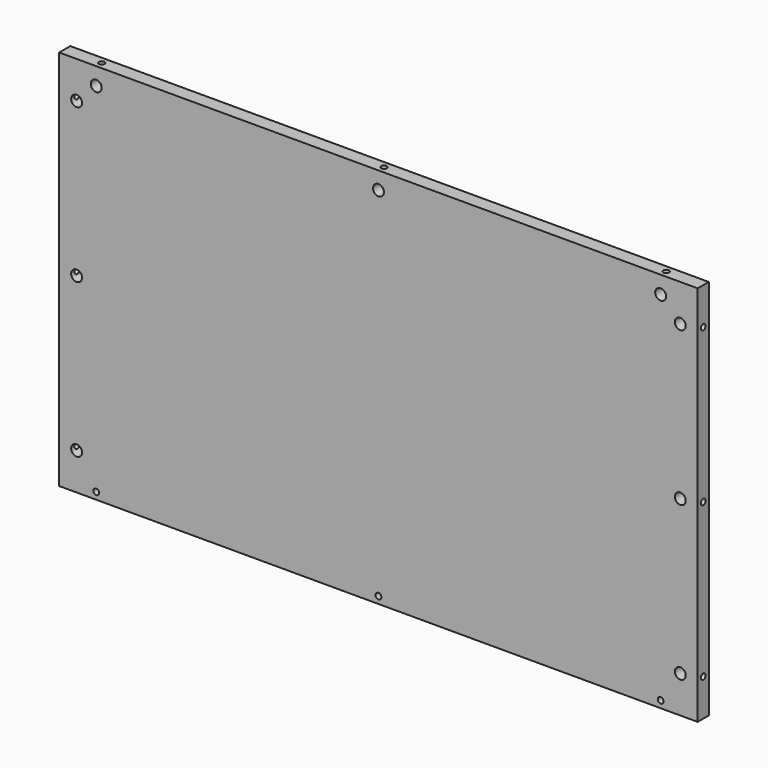
from build123d import *

# Parameters (mm, degrees)
F0_W      = 876.3
F0_H      = 523.875
F1_DEPTH  = 19.05
F3_D      = 15.0114
F3_DEPTH  = 14.224
F3_TIP    = 4.5098795482
F4_D      = 8.001
F4_DEPTH  = 14.224
F4_TIP    = 2.4037429064
F6_D      = 8.001
F6_DEPTH  = 25.4
F6_TIP    = 2.4037429064
F8_D      = 8.001
F8_DEPTH  = 25.4
F8_TIP    = 2.4037429064
F10_D     = 8.001
F10_DEPTH = 25.4
F10_TIP   = 2.4037429064


with BuildPart() as f1:
    # F0 (on Front) → F1 (new body)
    with BuildSketch(Plane.XZ):
        Rectangle(F0_W, F0_H)
    extrude(amount=F1_DEPTH)

    # F3
    with Locations(Plane.XZ.offset(19.05)):
        with Locations((-387.35, 238.0615), (-414.274, 211.1375), (-414.274, 0), (-414.274, -211.1375), (0, 238.0615), (387.35, 238.0615), (414.274, 211.1375), (414.274, 0), (414.274, -211.1375)):
            Hole(F3_D / 2, depth=F3_DEPTH)
            with Locations((0, 0, -(F3_DEPTH + F3_TIP / 2))):  # 118° drill point
                Cone(0, F3_D / 2, F3_TIP, mode=Mode.SUBTRACT)

    # F4
    with Locations(Plane.XZ.offset(19.05)):
        with Locations((-387.35, -252.4125), (0, -252.4125), (387.35, -252.4125)):
            Hole(F4_D / 2, depth=F4_DEPTH)
            with Locations((0, 0, -(F4_DEPTH + F4_TIP / 2))):  # 118° drill point
                Cone(0, F4_D / 2, F4_TIP, mode=Mode.SUBTRACT)

    # F6
    with Locations(Plane.YZ.offset(438.15)):
        with Locations((-9.525, 211.1375), (-9.525, 0), (-9.525, -211.1375)):
            Hole(F6_D / 2, depth=F6_DEPTH)
            with Locations((0, 0, -(F6_DEPTH + F6_TIP / 2))):  # 118° drill point
                Cone(0, F6_D / 2, F6_TIP, mode=Mode.SUBTRACT)

    # F8
    with Locations(Plane(origin=(-438.15, 0, 0), x_dir=(0, -1, 0), z_dir=(-1, 0, 0))):
        with Locations((9.525, 211.1375), (9.525, 0), (9.525, -211.1375)):
            Hole(F8_D / 2, depth=F8_DEPTH)
            with Locations((0, 0, -(F8_DEPTH + F8_TIP / 2))):  # 118° drill point
                Cone(0, F8_D / 2, F8_TIP, mode=Mode.SUBTRACT)

    # F10
    with Locations(Plane.XY.offset(261.9375)):
        with Locations((-387.35, -9.525), (0, -9.525), (387.35, -9.525)):
            Hole(F10_D / 2, depth=F10_DEPTH)
            with Locations((0, 0, -(F10_DEPTH + F10_TIP / 2))):  # 118° drill point
                Cone(0, F10_D / 2, F10_TIP, mode=Mode.SUBTRACT)


solid = f1.part
